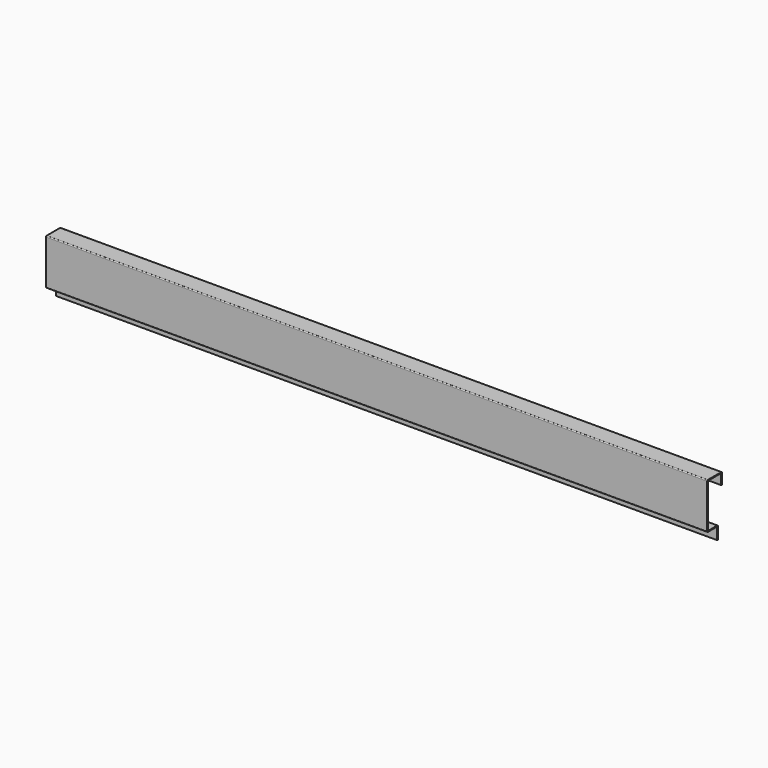
from build123d import *

# Parameters (mm, degrees)
F1_DEPTH = 1440
F3_D     = 5
F4_R     = 2


# Not quite as in the source:
# - a feature names something its author has since deleted; it is built from what else it names


with BuildPart() as f1:
    # F0 (on Right) → F1 (new body)
    with BuildSketch(Plane.YZ):
        Polygon((-18.8378913403, 177.8021101952), (-18.8378913403, 154.8021101952), (-16.8378913403, 154.8021101952), (-16.8378913403, 179.8021101952), (-56.8378913403, 179.8021101952), (-56.8378913403, 79.8021101952), (-29.8378913403, 79.8021101952), (-29.8378913403, 53.8021101952), (-27.8378913403, 53.8021101952), (-27.8378913403, 81.8021101952), (-54.8378913403, 81.8021101952), (-54.8378913403, 177.8021101952), align=None)
    extrude(amount=F1_DEPTH)

    # F3 (through all)
    with Locations(Plane.XZ.offset(29.8378913403)):
        with Locations((1340, 66.8021101952), (100, 66.8021101952)):
            Hole(F3_D / 2)

    # F4
    f4_edges = [f1.edges().sort_by_distance(p)[0] for p in [
        (720, -56.837891, 179.80211),
        (720, -16.837891, 179.80211),
        (720, -56.837891, 79.80211),
        (720, -27.837891, 81.80211),
        (720, -54.837891, 81.80211),
        (720, -29.837891, 79.80211),
        (720, -18.837891, 177.80211),
        (720, -54.837891, 177.80211),
    ]]
    fillet(f4_edges, radius=F4_R)


solid = f1.part
